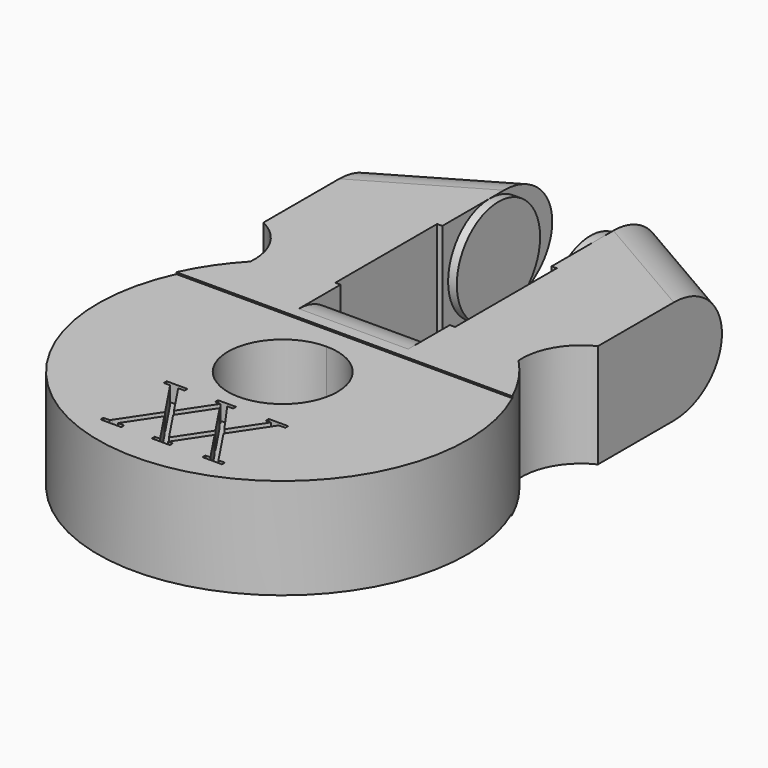
from build123d import *

# Parameters (mm, degrees)
F1_DEPTH  = 6
F2_R      = 3
F3_DEPTH  = 0.5
F4_R      = 3
F5_DEPTH  = 0.5
F6_R      = 2.99999
F7_R      = 2.99999
F9_DEPTH  = 1.1
F11_DEPTH = 1.2
F12_R     = 2.99999
F14_DEPTH = 13.4
F16_DEPTH = 0.1
F18_DEPTH = 0.1


# Not quite as in the source:
# - a fillet or chamfer is up to 0.001 mm smaller than in the source, because OpenCascade refuses the exact size


with BuildPart() as f1:
    # F0 (on Top) → F1 (new body)
    with BuildSketch(Plane.XY):
        with BuildLine():
            Line((-3.15, 8.1), (-3.15, 10.1734949747))
            ThreePointArc((-3.15, 10.1734949747), (-5.6194604457, 9.046776459), (-7.7238904562, 7.3323949854))
            ThreePointArc((-7.7238904562, 7.3323949854), (0, -10.65), (7.7238904562, 7.3323949854))
            ThreePointArc((7.7238904562, 7.3323949854), (5.6194604457, 9.046776459), (3.15, 10.1734949747))
            Line((3.15, 10.1734949747), (3.15, 8.1))
            Line((3.15, 8.1), (0, 8.1))
            Line((0, 8.1), (-3.15, 8.1))
        make_face()
        with BuildLine():
            ThreePointArc((3.15, 0), (-2.2273863607, -2.2273863607), (0, 3.15))
            ThreePointArc((0, 3.15), (2.2273863607, 2.2273863607), (3.15, 0))
        make_face(mode=Mode.SUBTRACT)
        with BuildLine():
            ThreePointArc((-7.7238904562, 7.3323949854), (-5.6194604457, 9.046776459), (-3.15, 10.1734949747))
            Line((-3.15, 10.1734949747), (-3.15, 23.35))
            Line((-3.15, 23.35), (-9.6377339195, 19.5871143267))
            Line((-9.6377339195, 19.5871143267), (-9.6377339195, 10.6575252249))
            ThreePointArc((-9.6377339195, 10.6575252249), (-8.1670066914, 9.2906908645), (-7.7238904562, 7.3323949854))
        make_face()
        with BuildLine():
            ThreePointArc((3.15, 10.1734949747), (5.6194604457, 9.046776459), (7.7238904562, 7.3323949854))
            ThreePointArc((7.7238904562, 7.3323949854), (8.1670066914, 9.2906908645), (9.6377339195, 10.6575252249))
            Line((9.6377339195, 10.6575252249), (9.6377339195, 19.5871143267))
            Line((9.6377339195, 19.5871143267), (3.15, 23.35))
            Line((3.15, 23.35), (3.15, 10.1734949747))
        make_face()
    extrude(amount=F1_DEPTH)

    # F2 (on face) → F3 (join)
    with BuildSketch(Plane.YZ.offset(-3.15)):
        with Locations((18.85, 3)):
            Circle(F2_R)
    extrude(amount=F3_DEPTH)

    # F4 (on face) → F5 (join)
    with BuildSketch(Plane(origin=(3.15, 0, 0), x_dir=(0, -1, 0), z_dir=(-1, 0, 0))):
        with Locations((-18.85, 3)):
            Circle(F4_R)
    extrude(amount=F5_DEPTH)

    # F6 (radius 3 in the source; OpenCascade refuses exactly that, so slightly less here)
    f6_edges = [f1.edges().sort_by_distance(p)[0] for p in [
        (-6.393867, 21.468557, 0),
        (-6.393867, 21.468557, 6),
    ]]
    fillet(f6_edges, radius=F6_R)

    # F7 (radius 3 in the source; OpenCascade refuses exactly that, so slightly less here)
    f7_edges = [f1.edges().sort_by_distance(p)[0] for p in [
        (6.393867, 21.468557, 0),
        (6.393867, 21.468557, 6),
    ]]
    fillet(f7_edges, radius=F7_R)

    # F8 (on face) → F9 (cut)
    with BuildSketch(Plane.XY.offset(6)):
        Polygon((-0.5410675658, -4.1934514275), (-0.2322952287, -4.1934514275), (-1.4496098506, -6.0194233604), (-2.6669244725, -4.1934514275), (-2.3, -4.1934514275), (-2.3, -3.9827399887), (-3.5, -3.9827399887), (-3.5, -4.1934514275), (-3.1341812573, -4.1934514275), (-2.8992197012, -4.5418942706), (-1.6819050793, -6.3678662034), (-3.0600394749, -8.4350677969), (-3.1399389263, -8.5422809794), (-3.5, -8.5422809794), (-3.5, -8.7529924182), (-2.3, -8.7529924182), (-2.3, -8.5422809794), (-2.6669244725, -8.5422809794), (-1.4496098506, -6.7163090465), (-0.2322952287, -8.5422809794), (-0.5410675658, -8.5422809794), (-0.5410675658, -8.7529924182), (0.5013382179, -8.7529924182), (0.5013382179, -8.5422809794), (0.2322952287, -8.5422809794), (1.4496098506, -6.7163090465), (2.6669244725, -8.5422809794), (2.3810260464, -8.5422809794), (2.3810260464, -8.7529924182), (3.4986780956, -8.7529924182), (3.5, -8.5422809794), (3.1424169429, -8.5422809794), (3.0600394749, -8.4350677969), (1.6819050793, -6.3678662034), (2.8992197012, -4.5418942706), (3.1315149299, -4.1934514275), (3.3579636365, -4.1934514275), (3.5, -4.1934514275), (3.4986780956, -3.9827399887), (2.3810260464, -3.9827399887), (2.3810260464, -4.1934514275), (2.6669244725, -4.1934514275), (1.4496098506, -6.0194233604), (0.1581401168, -4.1934514275), (0.5013382179, -4.1934514275), (0.5013382179, -3.9827399887), (-0.5410675658, -3.9827399887), align=None)
        Polygon((-1.2173146219, -6.3678662034), (0, -4.5418942706), (1.2173146219, -6.3678662034), (0, -8.1938381363), align=None, mode=Mode.SUBTRACT)
    extrude(amount=-F9_DEPTH, mode=Mode.SUBTRACT)

    # F10 (on face) → F11 (cut)
    with BuildSketch(Plane(origin=(0, 0, 0), x_dir=(1, 0, 0), z_dir=(0, 0, -1))):
        Polygon((-0.6402181378, 8.4924687258), (-0.3314458007, 8.4924687258), (-1.5487604226, 6.6664967929), (-2.7660750445, 8.4924687258), (-2.399150572, 8.4924687258), (-2.399150572, 8.7031801646), (-3.599150572, 8.7031801646), (-3.599150572, 8.4924687258), (-3.2333318293, 8.4924687258), (-2.9983702732, 8.1440258827), (-1.7810556513, 6.3180539499), (-3.1591900469, 4.2508523564), (-3.2390894983, 4.1436391739), (-3.599150572, 4.1436391739), (-3.599150572, 3.9329277351), (-2.399150572, 3.9329277351), (-2.399150572, 4.1436391739), (-2.7660750445, 4.1436391739), (-1.5487604226, 5.9696111068), (-0.3314458007, 4.1436391739), (-0.6402181378, 4.1436391739), (-0.6402181378, 3.9329277351), (0.4021876459, 3.9329277351), (0.4021876459, 4.1436391739), (0.1331446567, 4.1436391739), (1.3504592786, 5.9696111068), (2.5677739006, 4.1436391739), (2.2818754744, 4.1436391739), (2.2818754744, 3.9329277351), (3.3995275237, 3.9329277351), (3.400849428, 4.1436391739), (3.0432663709, 4.1436391739), (2.960888903, 4.2508523564), (1.5827545073, 6.3180539499), (2.8000691293, 8.1440258827), (3.032364358, 8.4924687258), (3.2588130645, 8.4924687258), (3.400849428, 8.4924687258), (3.3995275237, 8.7031801646), (2.2818754744, 8.7031801646), (2.2818754744, 8.4924687258), (2.5677739006, 8.4924687258), (1.3504592786, 6.6664967929), (0.0589895449, 8.4924687258), (0.4021876459, 8.4924687258), (0.4021876459, 8.7031801646), (-0.6402181378, 8.7031801646), align=None)
        Polygon((-1.3164651939, 6.3180539499), (-0.099150572, 8.1440258827), (1.1181640499, 6.3180539499), (-0.099150572, 4.492082017), align=None, mode=Mode.SUBTRACT)
    extrude(amount=-F11_DEPTH, mode=Mode.SUBTRACT)

    # F12 (radius 3 in the source; OpenCascade refuses exactly that, so slightly less here)
    f12_edges = [f1.edges().sort_by_distance(p)[0] for p in [
        (0, 8.1, 0),
        (0, 8.1, 6),
    ]]
    fillet(f12_edges, radius=F12_R)

    # F13 (on Top) → F14 (cut)
    with BuildSketch(Plane.XY):
        Polygon((-3.4496616572, 8.1000812352), (-3.1200703233, 8.1000812352), (-3.1314746011, 15.4313463718), (-3.4496616572, 15.4313463718), align=None)
        Polygon((3.1499122269, 8.1000812352), (3.4496616572, 8.1000812352), (3.4496616572, 15.4313463718), (3.1314746011, 15.4313463718), align=None)
    extrude(amount=F14_DEPTH, mode=Mode.SUBTRACT)

    # F15 (on face) → F16 (cut)
    with BuildSketch(Plane(origin=(0, 0, 0), x_dir=(1, 0, 0), z_dir=(0, 0, -1))):
        with BuildLine():
            Line((9.7270584918, -4.3366845744), (9.7615409984, -4.3366845744))
            ThreePointArc((9.7615409984, -4.3366845744), (0, 10.6815034411), (-9.7615409984, -4.3366845744))
            Line((-9.7615409984, -4.3366845744), (-9.7270584918, -4.3366845744))
            Line((-9.7270584918, -4.3366845744), (9.7270584918, -4.3366845744))
        make_face()
    extrude(amount=-F16_DEPTH, mode=Mode.SUBTRACT)

    # F17 (on face) → F18 (cut)
    with BuildSketch(Plane.XY.offset(6)):
        with BuildLine():
            Line((9.646881219, 4.4377580388), (-9.6813637257, 4.4377580388))
            ThreePointArc((-9.6813637257, 4.4377580388), (0, -10.65), (9.6813637257, 4.4377580388))
            Line((9.6813637257, 4.4377580388), (9.646881219, 4.4377580388))
        make_face()
    extrude(amount=-F18_DEPTH, mode=Mode.SUBTRACT)


solid = f1.part
